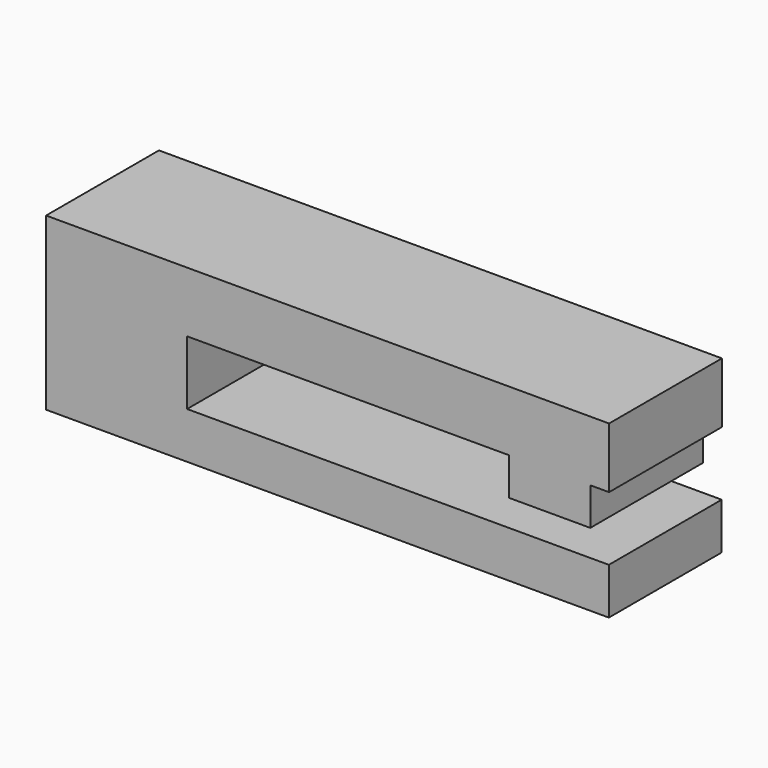
from build123d import *

# Parameters (mm, degrees)
F0_W     = 25.3896806389
F0_H     = 11.52669359
F0_W_2   = 14.6422572434
F0_H_2   = 6.7579634488
F1_DEPTH = 25.4


with BuildPart() as f1:
    # F0 (on Front) → F1 (new body)
    with BuildSketch(Plane.XZ):
        Polygon((52.3586980999, 30.7845659554), (-49.0107499063, 30.7845659554), (-49.0107499063, 19.8967363685), (-23.6210692674, 19.8967363685), (34.3374609947, 19.8967363685), (48.9797182381, 19.8967363685), (52.3586980999, 19.8967363685), align=None)
        with Locations((-36.3159095868, 14.1333895735)):
            Rectangle(F0_W, F0_H)
        Polygon((-23.6210692674, 8.3700427786), (-49.0107499063, 8.3700427786), (-49.0107499063, 0), (52.3202158511, 0), (52.3202158511, 8.3700427786), align=None)
        with Locations((41.6585896164, 16.5177546442)):
            Rectangle(F0_W_2, F0_H_2)
    extrude(amount=F1_DEPTH)


solid = f1.part
